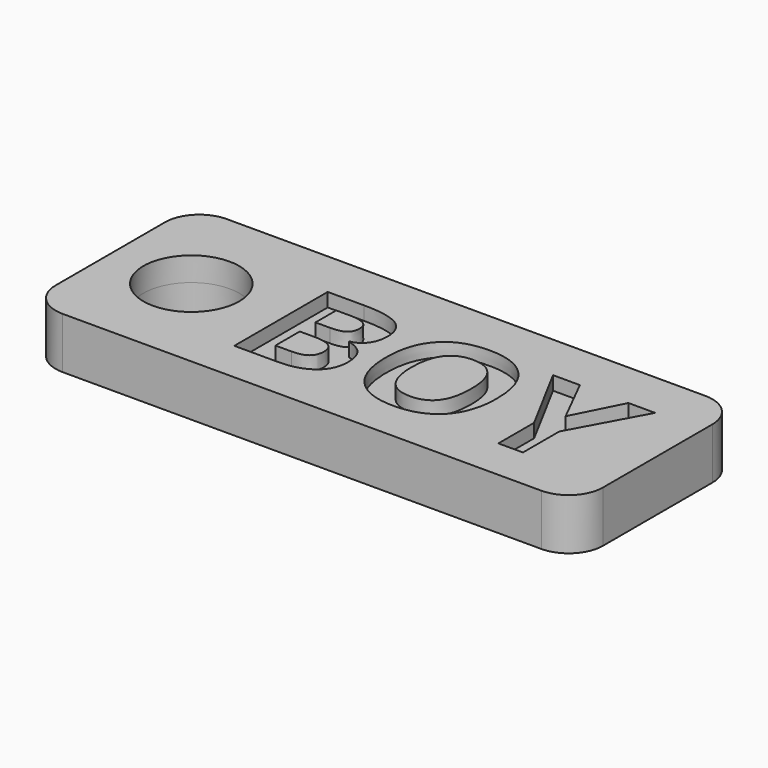
from build123d import *

# Parameters (mm, degrees)
F0_W         = 160
F0_H         = 60
F1_DEPTH     = 8
F2_R         = 14
F3_DEPTH     = 25
F4_DEPTH     = 7
F5_R         = 10
F7_TEXT_SIZE = 47.8092787994
F8_DEPTH     = 4


# Not quite as in the source:
# - Text() gives the source's letters only with a copy of the font that has no kerning and outlines rounded to 1/6400 em; it was checked with that copy


with BuildPart() as f1:
    # F0 (on Top) → F1 (new body)
    with BuildSketch(Plane.XY):
        Rectangle(F0_W, F0_H)
    extrude(amount=F1_DEPTH)

    # F2 (on face) → F3 (cut)
    with BuildSketch(Plane.XY.offset(8)):
        with Locations((-56.340161711, 0)):
            Circle(F2_R)
    extrude(amount=-F3_DEPTH, mode=Mode.SUBTRACT)

    # F4 (add): a face of the model
    f4_faces = [f1.faces().sort_by_distance(p)[0] for p in [
        (3.8613779242, 0, 8),
    ]]
    extrude(f4_faces, amount=F4_DEPTH)

    # F5
    f5_edges = [f1.edges().sort_by_distance(p)[0] for p in [
        (-80, -30, 7.5),
        (80, -30, 7.5),
        (80, 30, 7.5),
        (-80, 30, 7.5),
    ]]
    fillet(f5_edges, radius=F5_R)

    # F7 (on face) → F8 (cut)
    with BuildSketch(Plane.XY.offset(15)):
        with Locations((-33.7731949985, -17.8608242422)):
            Text('BOY', F7_TEXT_SIZE, font='Open Sans', font_style=FontStyle.BOLD, text_align=(TextAlign.LEFT, TextAlign.BOTTOM))
    extrude(amount=-F8_DEPTH, mode=Mode.SUBTRACT)


solid = f1.part
